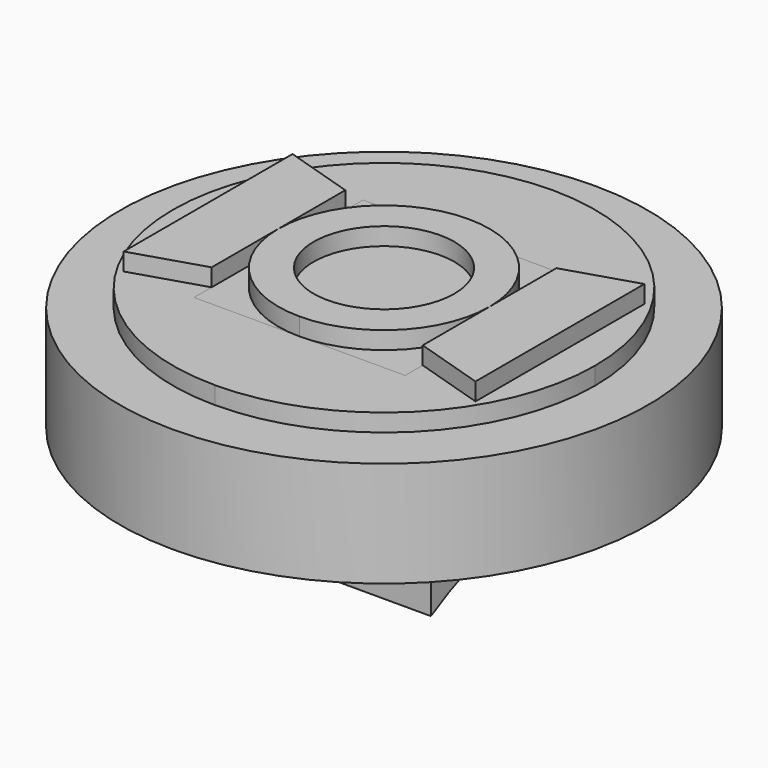
from build123d import *

# Parameters (mm, degrees)
F1_DEPTH  = 3
F2_DEPTH  = 3.5
F3_DEPTH  = 4
F0_W      = 3
F0_H      = 2
F7_DEPTH  = 6
F8_R      = 2
F9_DEPTH  = 0.5
F11_DEPTH = 3.5
F13_SCALE = 1.2
F14_ANGLE = 90
F15_W     = 12
F15_H     = 11
F16_DEPTH = 11
F17_R     = 11
F18_DEPTH = 12
F20_DEPTH = 0.6


# Not quite as in the source:
# - a feature of the source that left no trace in its solid (it failed there, or was rolled back) is left out


with BuildPart() as f1:
    # F0 (on Top) → F1 (new body)
    with BuildSketch(Plane.XY):
        with BuildLine():
            ThreePointArc((0, -7.5), (5.3033008589, -5.3033008589), (7.5, 0))
            Line((7.5, 0), (6, 0))
            ThreePointArc((6, 0), (4.2426406871, -4.2426406871), (0, -6))
            Line((0, -6), (0, -7.5))
        make_face()
        with BuildLine():
            ThreePointArc((-7.5, 0), (-5.3033008589, -5.3033008589), (0, -7.5))
            Line((0, -7.5), (0, -6))
            ThreePointArc((0, -6), (-4.2426406871, -4.2426406871), (-6, 0))
            Line((-6, 0), (-7.5, 0))
        make_face()
        with BuildLine():
            Line((0, 6), (0, 7.5))
            ThreePointArc((0, 7.5), (-5.3033008589, 5.3033008589), (-7.5, 0))
            Line((-7.5, 0), (-6, 0))
            ThreePointArc((-6, 0), (-4.2426406871, 4.2426406871), (0, 6))
        make_face()
        with BuildLine():
            Line((6, 0), (7.5, 0))
            ThreePointArc((7.5, 0), (5.3033008589, 5.3033008589), (0, 7.5))
            Line((0, 7.5), (0, 6))
            ThreePointArc((0, 6), (4.2426406871, 4.2426406871), (6, 0))
        make_face()
    extrude(amount=F1_DEPTH)

    # F0 (on Top) → F2 (join)
    with BuildSketch(Plane.XY):
        with BuildLine():
            ThreePointArc((0, -6), (4.2426406871, -4.2426406871), (6, 0))
            Line((6, 0), (3, 0))
            Line((3, 0), (3, -3))
            Line((3, -3), (3, -5))
            Line((3, -5), (0, -5))
            Line((0, -5), (0, -6))
        make_face()
        with BuildLine():
            Line((3, 0), (6, 0))
            ThreePointArc((6, 0), (4.2426406871, 4.2426406871), (0, 6))
            Line((0, 6), (0, 5))
            Line((0, 5), (3, 5))
            Line((3, 5), (3, 3))
            Line((3, 3), (3, 0))
        make_face()
        with BuildLine():
            Line((0, 5), (0, 6))
            ThreePointArc((0, 6), (-4.2426406871, 4.2426406871), (-6, 0))
            Line((-6, 0), (-3, 0))
            Line((-3, 0), (-3, 3))
            Line((-3, 3), (-3, 5))
            Line((-3, 5), (0, 5))
        make_face()
        with BuildLine():
            ThreePointArc((-6, 0), (-4.2426406871, -4.2426406871), (0, -6))
            Line((0, -6), (0, -5))
            Line((0, -5), (-3, -5))
            Line((-3, -5), (-3, -3))
            Line((-3, -3), (-3, 0))
            Line((-3, 0), (-6, 0))
        make_face()
    extrude(amount=F2_DEPTH)

    # F0 (on Top) → F3, piece 2 (join)
    with BuildSketch(Plane.XY):
        with Locations((1.5, -4)):
            Rectangle(F0_W, F0_H)
        with Locations((-1.5, -4)):
            Rectangle(F0_W, F0_H)
        with Locations((1.5, 4)):
            Rectangle(F0_W, F0_H)
        with Locations((-1.5, 4)):
            Rectangle(F0_W, F0_H)
    extrude(amount=F3_DEPTH)


with BuildPart() as f3:
    # F0 (on Top) → F3 (new body)
    with BuildSketch(Plane.XY):
        with BuildLine():
            ThreePointArc((0, -3), (2.1213203436, -2.1213203436), (3, 0))
            Line((3, 0), (0, 0))
            Line((0, 0), (0, -3))
        make_face()
        with BuildLine():
            ThreePointArc((-3, 0), (-2.1213203436, -2.1213203436), (0, -3))
            Line((0, -3), (0, 0))
            Line((0, 0), (-3, 0))
        make_face()
        with BuildLine():
            Line((0, 0), (0, 3))
            ThreePointArc((0, 3), (-2.1213203436, 2.1213203436), (-3, 0))
            Line((-3, 0), (0, 0))
        make_face()
        with BuildLine():
            Line((0, 0), (3, 0))
            ThreePointArc((3, 0), (2.1213203436, 2.1213203436), (0, 3))
            Line((0, 3), (0, 0))
        make_face()
    extrude(amount=F3_DEPTH)

    # F7 (add): a face of the model
    f7_faces = [f1.part.faces().sort_by_distance(p)[0] for p in [
        (-3, 0, 1.75),
    ]]
    extrude(f7_faces, amount=F7_DEPTH)

    # F8 (on face) → F9 (cut)
    with BuildSketch(Plane.XY.offset(4)):
        Circle(F8_R)
    extrude(amount=-F9_DEPTH, mode=Mode.SUBTRACT)


with BuildPart() as f11:
    # F10 (on Top) → F11 (new body)
    with BuildSketch(Plane.XY):
        with BuildLine():
            ThreePointArc((-24.2659887299, 12.9090552479), (-26.3873090735, 13.7877349043), (-27.2659887299, 15.9090552479))
            Line((-27.2659887299, 15.9090552479), (-27.2659887299, 12.9090552479))
            Line((-27.2659887299, 12.9090552479), (-24.2659887299, 12.9090552479))
        make_face()
    extrude(amount=-F11_DEPTH)


with BuildPart() as f11b:
    # F10 (on Top) → F11, piece 2 (new body)
    with BuildSketch(Plane.XY):
        with BuildLine():
            Line((-21.2659887299, 12.9090552479), (-21.2659887299, 15.9090552479))
            ThreePointArc((-21.2659887299, 15.9090552479), (-22.1446683863, 13.7877349043), (-24.2659887299, 12.9090552479))
            Line((-24.2659887299, 12.9090552479), (-21.2659887299, 12.9090552479))
        make_face()
    extrude(amount=-F11_DEPTH)


with BuildPart() as f11c:
    # F10 (on Top) → F11, piece 3 (new body)
    with BuildSketch(Plane.XY):
        with BuildLine():
            Line((-21.2659887299, 18.9090552479), (-24.2659887299, 18.9090552479))
            ThreePointArc((-24.2659887299, 18.9090552479), (-22.1446683863, 18.0303755915), (-21.2659887299, 15.9090552479))
            Line((-21.2659887299, 15.9090552479), (-21.2659887299, 18.9090552479))
        make_face()
    extrude(amount=-F11_DEPTH)


with BuildPart() as f11d:
    # F10 (on Top) → F11, piece 4 (new body)
    with BuildSketch(Plane.XY):
        with BuildLine():
            Line((-24.2659887299, 18.9090552479), (-27.2659887299, 18.9090552479))
            Line((-27.2659887299, 18.9090552479), (-27.2659887299, 15.9090552479))
            ThreePointArc((-27.2659887299, 15.9090552479), (-26.3873090735, 18.0303755915), (-24.2659887299, 18.9090552479))
        make_face()
    extrude(amount=-F11_DEPTH)


with BuildPart() as f1_1:
    # F13: moved
    add(f1.part.scale(F13_SCALE))


with BuildPart() as f3_1:
    # F13: moved
    add(f3.part.scale(F13_SCALE))


with BuildPart() as f1_2:
    # F14: moved
    add(f1_1.part.rotate(Axis((0, 0, 3.6), (0, 0, -1)), F14_ANGLE))

    # F15 (on face) → F16 (join)
    with BuildSketch(Plane(origin=(0, 0, 0), x_dir=(1, 0, 0), z_dir=(0, 0, -1))):
        Rectangle(F15_W, F15_H)
    extrude(amount=F16_DEPTH)

    # F17 (on face) → F18 (cut, through all)
    with BuildSketch(Plane.YZ.offset(6)):
        with Locations((0, -11.001)):
            Circle(F17_R)
    extrude(amount=-F18_DEPTH, mode=Mode.SUBTRACT)

    # F19 (on face) → F20 (cut, through all)
    with BuildSketch(Plane.XY.offset(4.8)):
        Polygon((3.6, 2.8490975965), (6, 3.6), (3.6, 3.6), align=None)
        Polygon((3.6, -3.6), (6, -3.6), (3.6, -2.8490975965), align=None)
        Polygon((-3.6, -2.8490975965), (-6, -3.6), (-3.6, -3.6), align=None)
        Polygon((-3.6, 3.6), (-6, 3.6), (-3.6, 2.8490975965), align=None)
    extrude(amount=-F20_DEPTH, mode=Mode.SUBTRACT)


solid = Compound([f3_1.part, f1_2.part])
